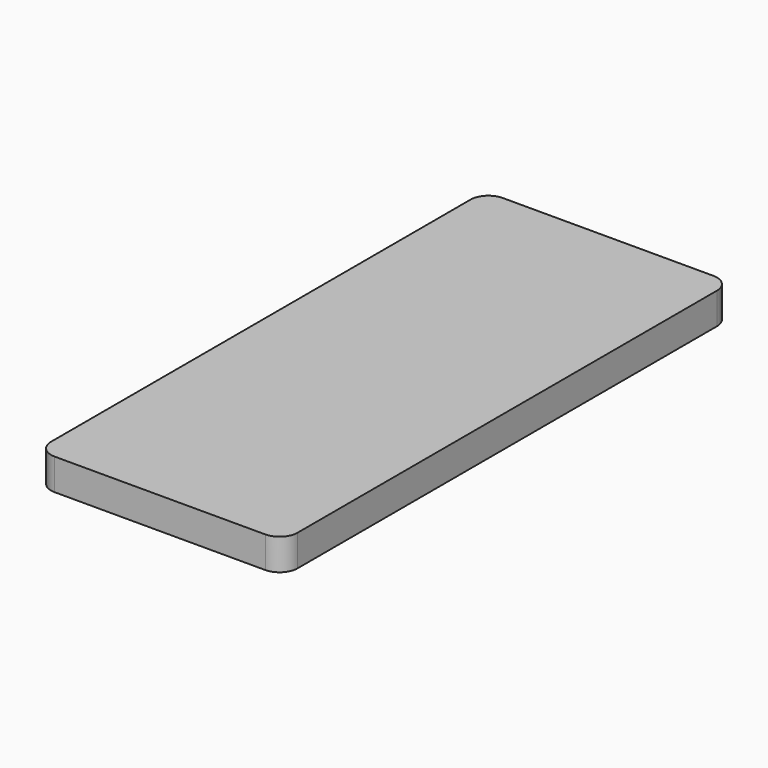
from build123d import *

# Parameters (mm, degrees)
F1_DEPTH = 7


# Not quite as in the source:
# - a feature of the source that left no trace in its solid (it failed there, or was rolled back) is left out


with BuildPart() as f1:
    # F0 (on Top) → F1 (new body)
    with BuildSketch(Plane.XY):
        with BuildLine():
            Line((23.5, 62.5), (-23.5, 62.5))
            ThreePointArc((-23.5, 62.5), (-26.3284271247, 61.3284271247), (-27.5, 58.5))
            Line((-27.5, 58.5), (-27.5, -58.5))
            ThreePointArc((-27.5, -58.5), (-26.3284271247, -61.3284271247), (-23.5, -62.5))
            Line((-23.5, -62.5), (23.5, -62.5))
            ThreePointArc((23.5, -62.5), (26.3284271247, -61.3284271247), (27.5, -58.5))
            Line((27.5, -58.5), (27.5, 58.5))
            ThreePointArc((27.5, 58.5), (26.3284271247, 61.3284271247), (23.5, 62.5))
        make_face()
    extrude(amount=F1_DEPTH)


solid = f1.part
